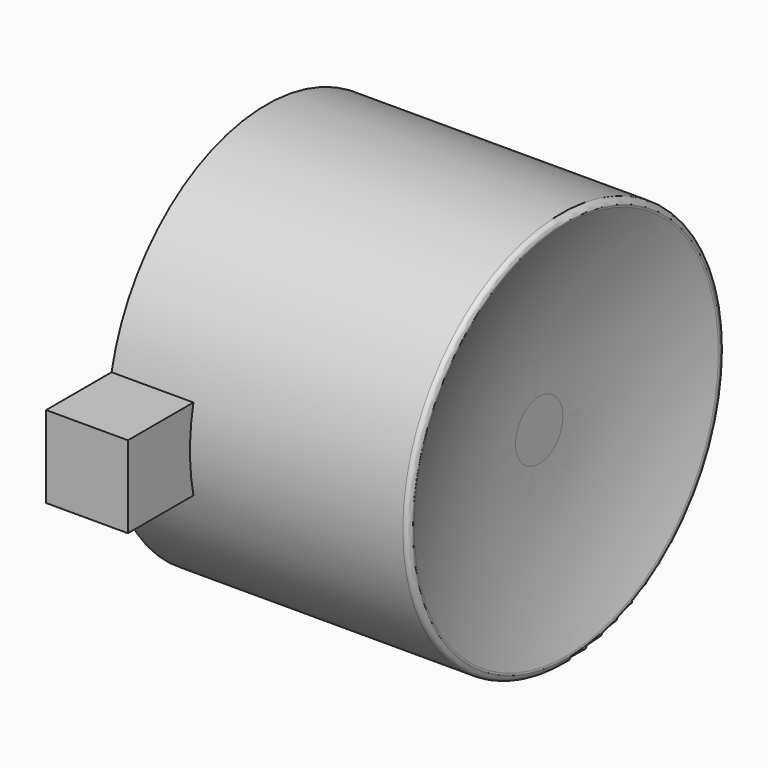
from build123d import *

# Parameters (mm, degrees)
F0_R     = 3.625
F1_DEPTH = 2.75
F2_T     = -1.25
F4_DEPTH = 1.5
F5_R     = 3.5
F6_DEPTH = 0.5
F8_R     = 0.1


# Not quite as in the source:
# - a fillet or chamfer that OpenCascade refuses, or shapes differently, is made with other operations: its cross-section is extruded or revolved along the edge and cut away or added


with BuildPart() as f1:
    # F0 (on Right) → F1 (new body, symmetric)
    with BuildSketch(Plane.YZ):
        Circle(F0_R)
    extrude(amount=F1_DEPTH, both=True)

    # F2
    f2_openings = [f1.faces().sort_by_distance(p)[0] for p in [
        (-2.75, 0, 0),
    ]]
    offset(amount=F2_T, openings=f2_openings)

    # F3 (on face) → F4 (join)
    with BuildSketch(Plane(origin=(-2.75, 0, 0), x_dir=(0, -1, 0), z_dir=(-1, 0, 0))):
        with BuildLine():
            Line((3.5465652398, -0.75), (5.0465652398, -0.75))
            Line((5.0465652398, -0.75), (5.0465652398, 0.75))
            Line((5.0465652398, 0.75), (3.5465652398, 0.75))
            ThreePointArc((3.5465652398, 0.75), (3.625, 0), (3.5465652398, -0.75))
        make_face()
        with BuildLine():
            Line((-3.5465652398, 0.75), (-5.0465652398, 0.75))
            Line((-5.0465652398, 0.75), (-5.0465652398, -0.75))
            Line((-5.0465652398, -0.75), (-3.5465652398, -0.75))
            ThreePointArc((-3.5465652398, -0.75), (-3.625, 0), (-3.5465652398, 0.75))
        make_face()
    extrude(amount=-F4_DEPTH)

    # F5 (on face) → F6 (cut)
    with BuildSketch(Plane.YZ.offset(2.75)):
        Circle(F5_R)
    extrude(amount=-F6_DEPTH, mode=Mode.SUBTRACT)

    # F7: fillet of radius 9 on 1 edges, made by hand

    # F7_s1 → F7_t2 (revolve)
    with BuildSketch(Plane.XY):
        with BuildLine():
            ThreePointArc((2.75, 3.5), (2.3758803254, 2.0419601084), (2.25, 0.5419601084))
            Line((2.25, 0.5419601084), (2.25, 3.5))
            Line((2.25, 3.5), (2.75, 3.5))
        make_face()
    revolve(axis=Axis((2.25, 0, 0), (1, 0, 0)))

    # F8
    f8_edges = [f1.edges().sort_by_distance(p)[0] for p in [
        (2.75, -3.5, 0),
        (2.75, -3.625, 0),
    ]]
    fillet(f8_edges, radius=F8_R)


solid = f1.part
